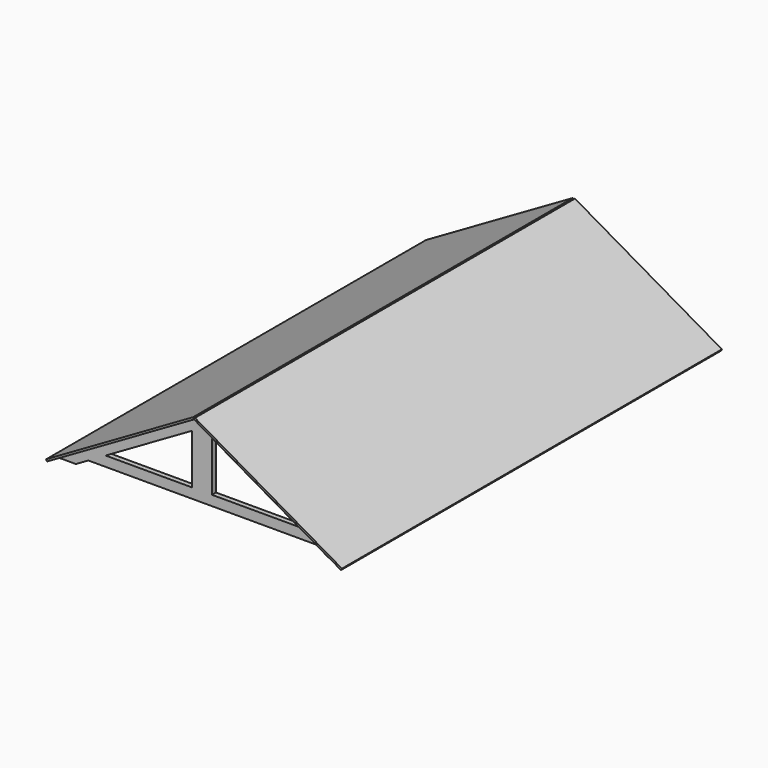
from build123d import *

# Parameters (mm, degrees)
F1_DEPTH       = 25
F7_W           = 1697.3335705802
F7_H           = 4750
F8_DEPTH       = 19
F11_DEPTH      = 725
F11_DEPTH_BACK = 725


with BuildPart() as f1:
    # F0 (on Front) → F1 (new body, symmetric)
    with BuildSketch(Plane.XZ):
        Polygon((-1261.2737367808, -71.7494753836), (-1137, 0), (-963.7949192431, 100), (-100, 598.7122291496), (0, 656.4472560686), (0, 771.9173099065), (-1337, 0), (-1461.2737367808, -71.7494753836), align=None)
        Polygon((-963.7949192431, 100), (-1137, 0), (1137, 0), (963.7949192431, 100), (100, 100), (0, 100), (-100, 100), align=None)
        Polygon((963.7949192431, 100), (1137, 0), (1261.2737367808, -71.7494753836), (1461.2737367808, -71.7494753836), (1337, 0), (0, 771.9173099065), (0, 656.4472560686), (100, 598.7122291496), align=None)
        Polygon((0, 656.4472560686), (-100, 598.7122291496), (-100, 100), (0, 100), align=None)
        Polygon((100, 598.7122291496), (0, 656.4472560686), (0, 100), (100, 100), align=None)
    extrude(amount=F1_DEPTH, both=True)


with BuildPart() as f3_1:
    # F3: instance of F1
    add(f1.part.mirror(Plane.XZ.offset(750)))


with BuildPart() as f5_1:
    # F5: instance of F3_1
    add(f3_1.part.mirror(Plane.XZ.offset(2250)))


with BuildPart() as f5_2:
    # F5: instance of F1
    add(f1.part.mirror(Plane.XZ.offset(2250)))


with BuildPart() as f8:
    # F7 (on face) → F8 (new body)
    with BuildSketch(Plane(origin=(-334.25, 0, 578.9379824299), x_dir=(0.8660254038, 0, 0.5), z_dir=(-0.5, 0, 0.8660254038))):
        with Locations((-462.7081303369, -2250)):
            Rectangle(F7_W, F7_H)
    extrude(amount=F8_DEPTH)


with BuildPart() as f9_1:
    # F9: instance of F8
    add(f8.part.mirror(Plane.YZ))


with BuildPart() as f11:
    # F10 (on offset) → F11 (new body, two sides)
    with BuildSketch(Plane.XZ.offset(750)) as f11_sk:
        Polygon((-1302.5155067444, 0), (-1137, 0), (1136.1624002457, 0), (1303.759932518, 0), (1303.759932518, 20), (1136.1624002457, 20), (-1137, 20), (-1302.5155067444, 20), align=None)
    extrude(amount=F11_DEPTH)
    extrude(f11_sk.sketch, amount=-F11_DEPTH_BACK)


solid = Compound([f1.part, f3_1.part, f5_1.part, f5_2.part, f8.part, f9_1.part, f11.part])
